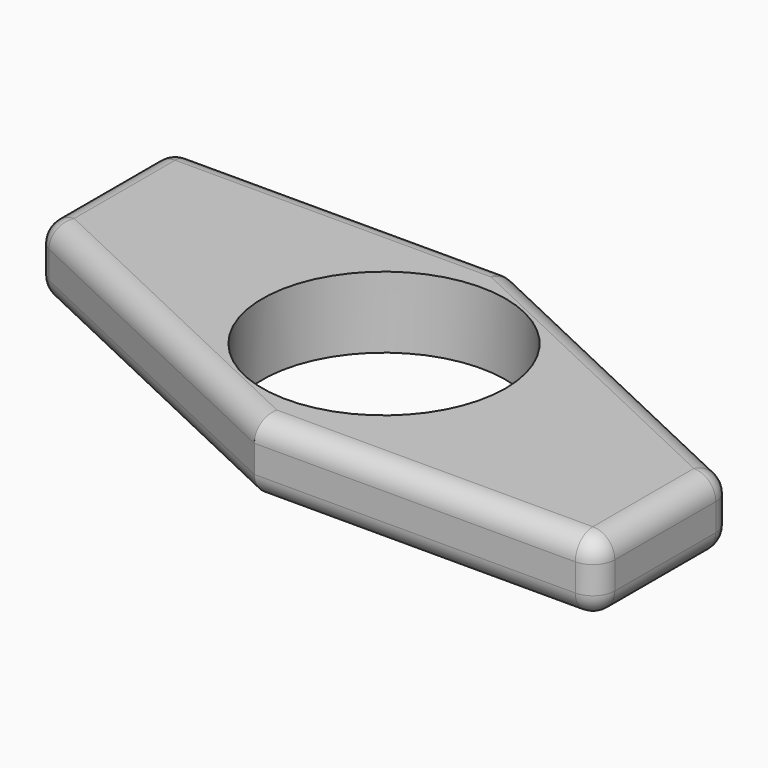
from build123d import *

# Parameters (mm, degrees)
F0_R         = 11.075
F1_DEPTH     = 6.5
F2_R         = 2
F3_T1_DEPTH  = 11.4968016823
F3_T3_DEPTH  = 2.5
F3_T5_DEPTH  = 32.8390350798
F3_S9_W      = 2
F3_S9_H      = 2
F3_T10_DEPTH = 2
F3_T16_DEPTH = 2
F3_T22_DEPTH = 2
F3_T28_DEPTH = 2
F3_T34_DEPTH = 2
F3_T38_ANGLE = 90


# Not quite as in the source:
# - a fillet or chamfer that OpenCascade refuses, or shapes differently, is made with other operations: its cross-section is extruded or revolved along the edge and cut away or added


with BuildPart() as f1:
    # F0 (on Top) → F1 (new body)
    with BuildSketch(Plane.XY):
        Polygon((31.2419999391, 0), (0, 14.7637501359), (-31.2419999391, 14.7637501359), (-31.2419999391, 0), (0, -14.7637501359), (31.2419999391, -14.7637501359), align=None)
        Circle(F0_R, mode=Mode.SUBTRACT)
    extrude(amount=F1_DEPTH)

    # F2
    f2_edges = [f1.edges().sort_by_distance(p)[0] for p in [
        (-31.242, 14.76375, 3.25),
        (-31.242, 0, 3.25),
        (15.621, -14.76375, 6.5),
        (15.621, -14.76375, 0),
        (15.621, 7.381875, 6.5),
        (-15.621, 14.76375, 6.5),
        (-15.621, 14.76375, 0),
        (-31.242, 7.381875, 0),
        (-31.242, 7.381875, 6.5),
        (-15.621, -7.381875, 6.5),
        (-15.621, -7.381875, 0),
        (31.242, -7.381875, 0),
    ]]
    fillet(f2_edges, radius=F2_R)

    # F3: fillet of radius 2 on 6 edges, made by hand

    # F3_s2 → F3_t1 (cut)
    with BuildSketch(Plane.XZ.offset(1.2669484536)):
        with BuildLine():
            ThreePointArc((31.2419999391, 4.5), (30.6562135015, 5.9142135624), (29.2419999391, 6.5))
            Line((29.2419999391, 6.5), (31.2419999391, 6.5))
            Line((31.2419999391, 6.5), (31.2419999391, 4.5))
        make_face()
    extrude(amount=F3_T1_DEPTH, mode=Mode.SUBTRACT)

    # F3_s4 → F3_t3 (cut)
    with BuildSketch(Plane.XY.offset(2)):
        with BuildLine():
            ThreePointArc((30.0965133896, 0.5413122474), (30.9315304806, -0.1966744002), (31.2419999391, -1.2669484536))
            Line((31.2419999391, -1.2669484536), (31.2419999391, 0))
            Line((31.2419999391, 0), (30.0965133896, 0.5413122474))
        make_face()
        with BuildLine():
            ThreePointArc((0.4057450927, 14.5720108369), (-0.0108878959, 14.7152266797), (-0.4487683579, 14.7637501359))
            Line((-0.4487683579, 14.7637501359), (0, 14.7637501359))
            Line((0, 14.7637501359), (0.4057450927, 14.5720108369))
        make_face()
        with BuildLine():
            ThreePointArc((31.2419999391, -12.7637501359), (30.6562135015, -14.1779636983), (29.2419999391, -14.7637501359))
            Line((29.2419999391, -14.7637501359), (31.2419999391, -14.7637501359))
            Line((31.2419999391, -14.7637501359), (31.2419999391, -12.7637501359))
        make_face()
    extrude(amount=F3_T3_DEPTH, mode=Mode.SUBTRACT)

    # F3_s6 → F3_t5 (cut)
    with BuildSketch(Plane(origin=(24.3933391217, -11.5273402623, 0), x_dir=(0, 0, 1), z_dir=(-0.9041303505, 0.4272567253, 0))):
        with BuildLine():
            ThreePointArc((2, 13.3483545851), (0.5857864376, 12.7625681475), (0, 11.3483545851))
            Line((0, 11.3483545851), (0, 13.3483545851))
            Line((0, 13.3483545851), (2, 13.3483545851))
        make_face()
    extrude(amount=F3_T5_DEPTH, mode=Mode.SUBTRACT)


with BuildPart() as f3_tool8:
    # F3_s9 → F3_t10 (new body)
    with BuildSketch(Plane.YZ.offset(29.2419999391)):
        with Locations((-13.7637501359, 1)):
            Rectangle(F3_S9_W, F3_S9_H)
    extrude(amount=F3_T10_DEPTH)

    # F3_s11 → F3_t12 (revolve, cut)
    with BuildSketch(Plane(origin=(29.2419999391, -12.7637501359, 2), x_dir=(0, 0.7071067812, 0.7071067812), z_dir=(0, 0.7071067812, -0.7071067812))):
        with BuildLine():
            ThreePointArc((0, -2), (2, 0), (0, 2))
            Line((0, 2), (0, -2))
        make_face()
    revolve(axis=Axis((29.2419999391, -12.7637501359, 2), (1, 0, 0)), mode=Mode.SUBTRACT)


with BuildPart() as f1_1:
    add(f1.part)

    # F3_t7: cut F3_tool8
    add(f3_tool8.part, mode=Mode.SUBTRACT)


with BuildPart() as f3_tool14:
    # F3_s15 → F3_t16 (new body)
    with BuildSketch(Plane.XY.offset(4.5)):
        Polygon((-0.4487683579, 12.7637501359), (0.4057450927, 14.5720108369), (0, 14.7637501359), (-0.4487683579, 14.7637501359), align=None)
    extrude(amount=F3_T16_DEPTH)

    # F3_s17 → F3_t18 (revolve, cut)
    with BuildSketch(Plane(origin=(-0.4487683579, 12.7637501359, 4.5), x_dir=(-0.218940231, -0.9757382719, 0), z_dir=(-0.9757382719, 0.218940231, 0))):
        with BuildLine():
            ThreePointArc((0, -2), (2, 0), (0, 2))
            Line((0, 2), (0, -2))
        make_face()
    revolve(axis=Axis((-0.4487683579, 12.7637501359, 4.5), (0, 0, 1)), mode=Mode.SUBTRACT)


with BuildPart() as f1_2:
    add(f1_1.part)

    # F3_t13: cut F3_tool14
    add(f3_tool14.part, mode=Mode.SUBTRACT)


with BuildPart() as f3_tool20:
    # F3_s21 → F3_t22 (new body)
    with BuildSketch(Plane.XY.offset(2)):
        Polygon((-0.4487683579, 12.7637501359), (-0.4487683579, 14.7637501359), (0, 14.7637501359), (0.4057450927, 14.5720108369), align=None)
    extrude(amount=-F3_T22_DEPTH)

    # F3_s23 → F3_t24 (revolve, cut)
    with BuildSketch(Plane(origin=(-0.4487683579, 12.7637501359, 2), x_dir=(-0.218940231, -0.9757382719, 0), z_dir=(0.9757382719, -0.218940231, 0))):
        with BuildLine():
            ThreePointArc((0, -2), (2, 0), (0, 2))
            Line((0, 2), (0, -2))
        make_face()
    revolve(axis=Axis((-0.4487683579, 12.7637501359, 2), (0, 0, -1)), mode=Mode.SUBTRACT)


with BuildPart() as f1_3:
    add(f1_2.part)

    # F3_t19: cut F3_tool20
    add(f3_tool20.part, mode=Mode.SUBTRACT)


with BuildPart() as f3_tool26:
    # F3_s27 → F3_t28 (new body)
    with BuildSketch(Plane.XY.offset(2)):
        Polygon((29.2419999391, -1.2669484536), (30.0965133896, 0.5413122474), (31.2419999391, 0), (31.2419999391, -1.2669484536), align=None)
    extrude(amount=-F3_T28_DEPTH)

    # F3_s29 → F3_t30 (revolve, cut)
    with BuildSketch(Plane(origin=(29.2419999391, -1.2669484536, 2), x_dir=(-0.8447652707, -0.5351370267, 0), z_dir=(0.5351370267, -0.8447652707, 0))):
        with BuildLine():
            ThreePointArc((0, -2), (2, 0), (0, 2))
            Line((0, 2), (0, -2))
        make_face()
    revolve(axis=Axis((29.2419999391, -1.2669484536, 2), (0, 0, -1)), mode=Mode.SUBTRACT)


with BuildPart() as f1_4:
    add(f1_3.part)

    # F3_t25: cut F3_tool26
    add(f3_tool26.part, mode=Mode.SUBTRACT)


with BuildPart() as f3_tool32:
    # F3_s33 → F3_t34 (new body)
    with BuildSketch(Plane.XY.offset(4.5)):
        Polygon((29.2419999391, -1.2669484536), (30.0965133896, 0.5413122474), (31.2419999391, 0), (31.2419999391, -1.2669484536), align=None)
    extrude(amount=F3_T34_DEPTH)

    # F3_s35 → F3_t36 (revolve, cut)
    with BuildSketch(Plane(origin=(29.2419999391, -1.2669484536, 4.5), x_dir=(-0.8447652707, -0.5351370267, 0), z_dir=(-0.5351370267, 0.8447652707, 0))):
        with BuildLine():
            ThreePointArc((0, -2), (2, 0), (0, 2))
            Line((0, 2), (0, -2))
        make_face()
    revolve(axis=Axis((29.2419999391, -1.2669484536, 4.5), (0, 0, 1)), mode=Mode.SUBTRACT)


with BuildPart() as f1_5:
    add(f1_4.part)

    # F3_t31: cut F3_tool32
    add(f3_tool32.part, mode=Mode.SUBTRACT)

    # F3_s37 → F3_t38 (revolve, cut)
    with BuildSketch(Plane.XY.offset(4.5)):
        with BuildLine():
            ThreePointArc((31.2419999391, -12.7637501359), (30.6562135015, -14.1779636983), (29.2419999391, -14.7637501359))
            Line((29.2419999391, -14.7637501359), (31.2419999391, -14.7637501359))
            Line((31.2419999391, -14.7637501359), (31.2419999391, -12.7637501359))
        make_face()
    revolve(axis=Axis((31.2419999391, -12.7637501359, 4.5), (-1, 0, 0)), revolution_arc=F3_T38_ANGLE, mode=Mode.SUBTRACT)


solid = f1_5.part
